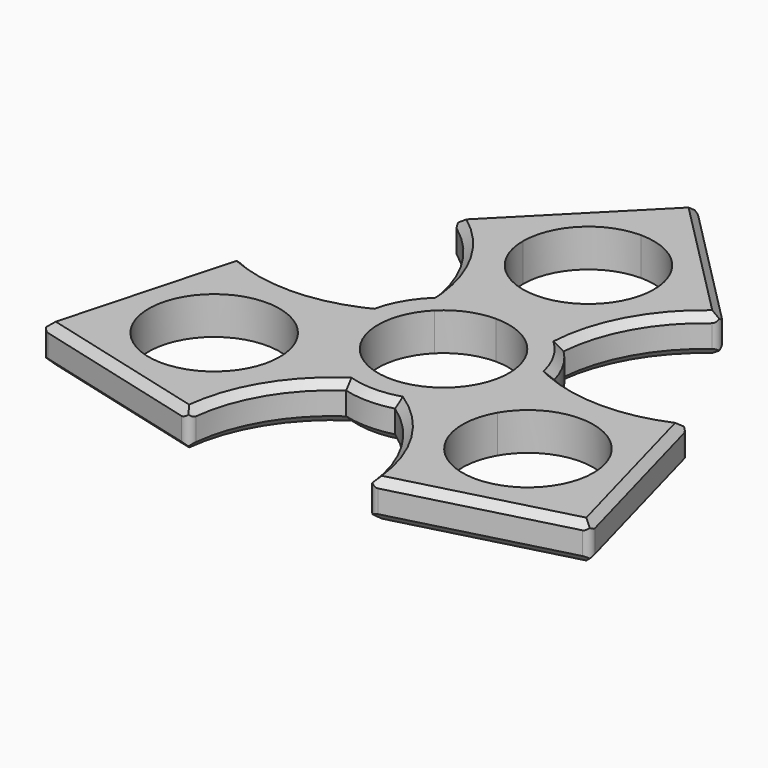
from build123d import *

# Parameters (mm, degrees)
F1_DEPTH    = 6.35
F2_C1_SIZE  = 1.27
F2_C2_SIZE  = 1.27
F2_C3_SIZE  = 1.27
F2_C4_SIZE  = 1.27
F2_C5_SIZE  = 1.2699
F2_C6_SIZE  = 1.2699
F2_C7_SIZE  = 1.27
F2_C8_SIZE  = 1.27
F2_C9_SIZE  = 1.27
F2_C10_SIZE = 1.27
F2_C11_SIZE = 1.27
F2_C12_SIZE = 1.27
F2_C13_SIZE = 1.27
F2_C14_SIZE = 1.27
F2_C15_SIZE = 1.2696
F3_C1_SIZE  = 1.27
F3_C2_SIZE  = 1.27
F3_C3_SIZE  = 1.27
F3_C4_SIZE  = 1.27
F3_C5_SIZE  = 1.27
F3_C6_SIZE  = 1.27
F3_C7_SIZE  = 1.2699
F3_C8_SIZE  = 1.27
F3_C9_SIZE  = 1.27
F3_C10_SIZE = 1.27
F3_C11_SIZE = 1.27
F3_C12_SIZE = 1.2696
F3_C13_SIZE = 1.27
F3_C14_SIZE = 1.27
F3_C15_SIZE = 1.27
F4_R        = 1.27


# Not quite as in the source:
# - a fillet or chamfer is up to 0.001 mm smaller than in the source, because OpenCascade refuses the exact size


with BuildPart() as f1:
    # F0 (on Top) → F1 (new body)
    with BuildSketch(Plane.XY):
        with BuildLine():
            ThreePointArc((-4.108752341, -15.3340724923), (-9.6640876855, -12.5944842771), (-13.7481532851, -7.9375))
            ThreePointArc((-13.7481532851, -7.9375), (-15.7391871743, -2.0721033015), (-15.3340724923, 4.108752341))
            ThreePointArc((-15.3340724923, 4.108752341), (-26.5599121407, 1.6434086068), (-37.7231270498, 4.3783726706))
            Line((-37.7231270498, 4.3783726706), (-46.1937950379, -26.67))
            Line((-46.1937950379, -26.67), (-15.0697815649, -34.8583726706))
            ThreePointArc((-15.0697815649, -34.8583726706), (-11.856722468, -23.8232629395), (-4.108752341, -15.3340724923))
        make_face()
        with BuildLine():
            ThreePointArc((-15.3855543073, -15.24), (-37.032166988, -18.0898306237), (-16.8607351888, -9.73455))
            ThreePointArc((-16.8607351888, -9.73455), (-15.7607416267, -12.3901693763), (-15.3855543073, -15.24))
        make_face(mode=Mode.SUBTRACT)
        with BuildLine():
            ThreePointArc((-11.2253201513, 11.2253201513), (-6.0750994888, 14.6665875786), (0, 15.875))
            Line((0, 15.875), (0, 19.4691))
            ThreePointArc((0, 19.4691), (-7.785882057, 22.694117943), (-11.0109, 30.48))
            Line((-11.0109, 30.48), (-22.6533454849, 30.48))
            ThreePointArc((-22.6533454849, 30.48), (-14.7031896726, 22.1798543327), (-11.2253201513, 11.2253201513))
        make_face()
        with BuildLine():
            ThreePointArc((15.875, 0), (15.3340724923, -4.108752341), (13.7481532851, -7.9375))
            ThreePointArc((13.7481532851, -7.9375), (9.6640876855, -12.5944842771), (4.108752341, -15.3340724923))
            ThreePointArc((4.108752341, -15.3340724923), (11.856722468, -23.8232629395), (15.0697815649, -34.8583726706))
            Line((15.0697815649, -34.8583726706), (46.1937950379, -26.67))
            Line((46.1937950379, -26.67), (37.7231270498, 4.3783726706))
            ThreePointArc((37.7231270498, 4.3783726706), (26.5599121407, 1.6434086068), (15.3340724923, 4.108752341))
            ThreePointArc((15.3340724923, 4.108752341), (15.7391871743, 2.0721033015), (15.875, 0))
        make_face()
        with BuildLine():
            ThreePointArc((37.4073543073, -15.24), (23.5466236836, -25.8757126807), (16.8607351888, -9.73455))
            ThreePointArc((16.8607351888, -9.73455), (29.2462849311, -4.6042873193), (37.4073543073, -15.24))
        make_face(mode=Mode.SUBTRACT)
        with BuildLine():
            ThreePointArc((7.785882057, 7.785882057), (10.1727451445, 4.2136890054), (11.0109, 0))
            ThreePointArc((11.0109, 0), (10.6357126807, -2.8498306237), (9.5357191185, -5.50545))
            Line((9.5357191185, -5.50545), (13.7481532851, -7.9375))
            ThreePointArc((13.7481532851, -7.9375), (15.3340724923, -4.108752341), (15.875, 0))
            ThreePointArc((15.875, 0), (15.7391871743, 2.0721033015), (15.3340724923, 4.108752341))
            ThreePointArc((15.3340724923, 4.108752341), (13.7481532851, 7.9375), (11.2253201513, 11.2253201513))
            Line((11.2253201513, 11.2253201513), (7.785882057, 7.785882057))
        make_face()
        with BuildLine():
            Line((13.7481532851, -7.9375), (9.5357191185, -5.50545))
            ThreePointArc((9.5357191185, -5.50545), (0, -11.0109), (-9.5357191185, -5.50545))
            Line((-9.5357191185, -5.50545), (-13.7481532851, -7.9375))
            ThreePointArc((-13.7481532851, -7.9375), (-9.6640876855, -12.5944842771), (-4.108752341, -15.3340724923))
            ThreePointArc((-4.108752341, -15.3340724923), (0, -15.875), (4.108752341, -15.3340724923))
            ThreePointArc((4.108752341, -15.3340724923), (9.6640876855, -12.5944842771), (13.7481532851, -7.9375))
        make_face()
        with BuildLine():
            Line((-13.7481532851, -7.9375), (-9.5357191185, -5.50545))
            ThreePointArc((-9.5357191185, -5.50545), (-10.9167002241, 1.4372108499), (-7.785882057, 7.785882057))
            Line((-7.785882057, 7.785882057), (-11.2253201513, 11.2253201513))
            ThreePointArc((-11.2253201513, 11.2253201513), (-13.7481532851, 7.9375), (-15.3340724923, 4.108752341))
            ThreePointArc((-15.3340724923, 4.108752341), (-15.7391871743, -2.0721033015), (-13.7481532851, -7.9375))
        make_face()
        with BuildLine():
            ThreePointArc((-7.785882057, 7.785882057), (-4.2136890054, 10.1727451445), (0, 11.0109))
            Line((0, 11.0109), (0, 15.875))
            ThreePointArc((0, 15.875), (-6.0750994888, 14.6665875786), (-11.2253201513, 11.2253201513))
            Line((-11.2253201513, 11.2253201513), (-7.785882057, 7.785882057))
        make_face()
        with BuildLine():
            ThreePointArc((0, 11.0109), (4.2136890054, 10.1727451445), (7.785882057, 7.785882057))
            Line((7.785882057, 7.785882057), (11.2253201513, 11.2253201513))
            ThreePointArc((11.2253201513, 11.2253201513), (6.0750994888, 14.6665875786), (0, 15.875))
            Line((0, 15.875), (0, 11.0109))
        make_face()
        with BuildLine():
            Line((0, 41.4909), (0, 53.34))
            Line((0, 53.34), (-22.6533454849, 30.48))
            Line((-22.6533454849, 30.48), (-11.0109, 30.48))
            ThreePointArc((-11.0109, 30.48), (-7.785882057, 38.265882057), (0, 41.4909))
        make_face()
        with BuildLine():
            Line((11.0109, 30.48), (22.6533454849, 30.48))
            Line((22.6533454849, 30.48), (0, 53.34))
            Line((0, 53.34), (0, 41.4909))
            ThreePointArc((0, 41.4909), (7.785882057, 38.265882057), (11.0109, 30.48))
        make_face()
        with BuildLine():
            ThreePointArc((0, 15.875), (6.0750994888, 14.6665875786), (11.2253201513, 11.2253201513))
            ThreePointArc((11.2253201513, 11.2253201513), (14.7031896726, 22.1798543327), (22.6533454849, 30.48))
            Line((22.6533454849, 30.48), (11.0109, 30.48))
            ThreePointArc((11.0109, 30.48), (7.785882057, 22.694117943), (0, 19.4691))
            Line((0, 19.4691), (0, 15.875))
        make_face()
    extrude(amount=F1_DEPTH)

    # F2: chamfer of 1.27 on 15 edges, made by hand

    # F2_c1
    f2_c1_edges = [f1.edges().sort_by_distance(p)[0] for p in [
        (-26.5599121407, 1.6434086068, 6.35),
    ]]
    chamfer(f2_c1_edges, length=F2_C1_SIZE)

    # F2_c2
    f2_c2_edges = [f1.edges().sort_by_distance(p)[0] for p in [
        (-42.128898124, -11.7705334612, 6.35),
    ]]
    chamfer(f2_c2_edges, length=F2_C2_SIZE)

    # F2_c3
    f2_c3_edges = [f1.edges().sort_by_distance(p)[0] for p in [
        (-30.0176601745, -30.9257564353, 6.35),
    ]]
    chamfer(f2_c3_edges, length=F2_C3_SIZE)

    # F2_c4
    f2_c4_edges = [f1.edges().sort_by_distance(p)[0] for p in [
        (-11.5338044819, -23.2648005925, 6.35),
    ]]
    chamfer(f2_c4_edges, length=F2_C4_SIZE)

    # F2_c5 (size 1.27 in the source; OpenCascade refuses exactly that, so slightly less here)
    f2_c5_edges = [f1.edges().sort_by_distance(p)[0] for p in [
        (0, -15.875, 6.35),
    ]]
    chamfer(f2_c5_edges, length=F2_C5_SIZE)

    # F2_c6 (size 1.27 in the source; OpenCascade refuses exactly that, so slightly less here)
    f2_c6_edges = [f1.edges().sort_by_distance(p)[0] for p in [
        (11.856722468, -23.8232629395, 6.35),
    ]]
    chamfer(f2_c6_edges, length=F2_C6_SIZE)

    # F2_c7
    f2_c7_edges = [f1.edges().sort_by_distance(p)[0] for p in [
        (31.2579807919, -30.5994422389, 6.35),
    ]]
    chamfer(f2_c7_edges, length=F2_C7_SIZE)

    # F2_c8
    f2_c8_edges = [f1.edges().sort_by_distance(p)[0] for p in [
        (41.7913207915, -10.5331780556, 6.35),
    ]]
    chamfer(f2_c8_edges, length=F2_C8_SIZE)

    # F2_c9
    f2_c9_edges = [f1.edges().sort_by_distance(p)[0] for p in [
        (25.9148105681, 1.6438326126, 6.35),
    ]]
    chamfer(f2_c9_edges, length=F2_C9_SIZE)

    # F2_c10
    f2_c10_edges = [f1.edges().sort_by_distance(p)[0] for p in [
        (13.7481532851, 7.9375, 6.35),
    ]]
    chamfer(f2_c10_edges, length=F2_C10_SIZE)

    # F2_c11
    f2_c11_edges = [f1.edges().sort_by_distance(p)[0] for p in [
        (14.7031896726, 22.1798543327, 6.35),
    ]]
    chamfer(f2_c11_edges, length=F2_C11_SIZE)

    # F2_c12
    f2_c12_edges = [f1.edges().sort_by_distance(p)[0] for p in [
        (10.8708680685, 42.3699627394, 6.35),
    ]]
    chamfer(f2_c12_edges, length=F2_C12_SIZE)

    # F2_c13
    f2_c13_edges = [f1.edges().sort_by_distance(p)[0] for p in [
        (-11.773660617, 41.4589344909, 6.35),
    ]]
    chamfer(f2_c13_edges, length=F2_C13_SIZE)

    # F2_c14
    f2_c14_edges = [f1.edges().sort_by_distance(p)[0] for p in [
        (-14.3810060862, 21.6209679799, 6.35),
    ]]
    chamfer(f2_c14_edges, length=F2_C14_SIZE)

    # F2_c15 (size 1.27 in the source; OpenCascade refuses exactly that, so slightly less here)
    f2_c15_edges = [f1.edges().sort_by_distance(p)[0] for p in [
        (-13.7481532851, 7.9375, 6.35),
    ]]
    chamfer(f2_c15_edges, length=F2_C15_SIZE)

    # F3: chamfer of 1.27 on 15 edges, made by hand

    # F3_c1
    f3_c1_edges = [f1.edges().sort_by_distance(p)[0] for p in [
        (-13.7481532851, 7.9375, 0),
    ]]
    chamfer(f3_c1_edges, length=F3_C1_SIZE)

    # F3_c2
    f3_c2_edges = [f1.edges().sort_by_distance(p)[0] for p in [
        (-14.7031896726, 22.1798543327, 0),
    ]]
    chamfer(f3_c2_edges, length=F3_C2_SIZE)

    # F3_c3
    f3_c3_edges = [f1.edges().sort_by_distance(p)[0] for p in [
        (-10.8708680685, 42.3699627394, 0),
    ]]
    chamfer(f3_c3_edges, length=F3_C3_SIZE)

    # F3_c4
    f3_c4_edges = [f1.edges().sort_by_distance(p)[0] for p in [
        (11.773660617, 41.4589344909, 0),
    ]]
    chamfer(f3_c4_edges, length=F3_C4_SIZE)

    # F3_c5
    f3_c5_edges = [f1.edges().sort_by_distance(p)[0] for p in [
        (14.3810060862, 21.6209679799, 0),
    ]]
    chamfer(f3_c5_edges, length=F3_C5_SIZE)

    # F3_c6
    f3_c6_edges = [f1.edges().sort_by_distance(p)[0] for p in [
        (-26.5599121407, 1.6434086068, 0),
    ]]
    chamfer(f3_c6_edges, length=F3_C6_SIZE)

    # F3_c7 (size 1.27 in the source; OpenCascade refuses exactly that, so slightly less here)
    f3_c7_edges = [f1.edges().sort_by_distance(p)[0] for p in [
        (13.7481532851, 7.9375, 0),
    ]]
    chamfer(f3_c7_edges, length=F3_C7_SIZE)

    # F3_c8
    f3_c8_edges = [f1.edges().sort_by_distance(p)[0] for p in [
        (-42.128898124, -11.7705334612, 0),
    ]]
    chamfer(f3_c8_edges, length=F3_C8_SIZE)

    # F3_c9
    f3_c9_edges = [f1.edges().sort_by_distance(p)[0] for p in [
        (-30.0176601745, -30.9257564353, 0),
    ]]
    chamfer(f3_c9_edges, length=F3_C9_SIZE)

    # F3_c10
    f3_c10_edges = [f1.edges().sort_by_distance(p)[0] for p in [
        (0, -15.875, 0),
    ]]
    chamfer(f3_c10_edges, length=F3_C10_SIZE)

    # F3_c11
    f3_c11_edges = [f1.edges().sort_by_distance(p)[0] for p in [
        (-11.5338044819, -23.2648005925, 0),
    ]]
    chamfer(f3_c11_edges, length=F3_C11_SIZE)

    # F3_c12 (size 1.27 in the source; OpenCascade refuses exactly that, so slightly less here)
    f3_c12_edges = [f1.edges().sort_by_distance(p)[0] for p in [
        (26.5599121407, 1.6434086068, 0),
    ]]
    chamfer(f3_c12_edges, length=F3_C12_SIZE)

    # F3_c13
    f3_c13_edges = [f1.edges().sort_by_distance(p)[0] for p in [
        (42.128844494, -11.7703368859, 0),
    ]]
    chamfer(f3_c13_edges, length=F3_C13_SIZE)

    # F3_c14
    f3_c14_edges = [f1.edges().sort_by_distance(p)[0] for p in [
        (30.0176601745, -30.9257564353, 0),
    ]]
    chamfer(f3_c14_edges, length=F3_C14_SIZE)

    # F3_c15
    f3_c15_edges = [f1.edges().sort_by_distance(p)[0] for p in [
        (11.5338044819, -23.2648005925, 0),
    ]]
    chamfer(f3_c15_edges, length=F3_C15_SIZE)

    # F4
    f4_edges = [f1.edges().sort_by_distance(p)[0] for p in [
        (46.193795, -26.67, 3.175),
        (37.723127, 4.378373, 3.175),
        (22.653345, 30.48, 3.175),
        (0, 53.34, 3.175),
        (-22.653345, 30.48, 3.175),
        (-37.723127, 4.378373, 3.175),
        (-46.193795, -26.67, 3.175),
        (-15.069782, -34.858373, 3.175),
        (15.069782, -34.858373, 3.175),
    ]]
    fillet(f4_edges, radius=F4_R)


solid = f1.part
